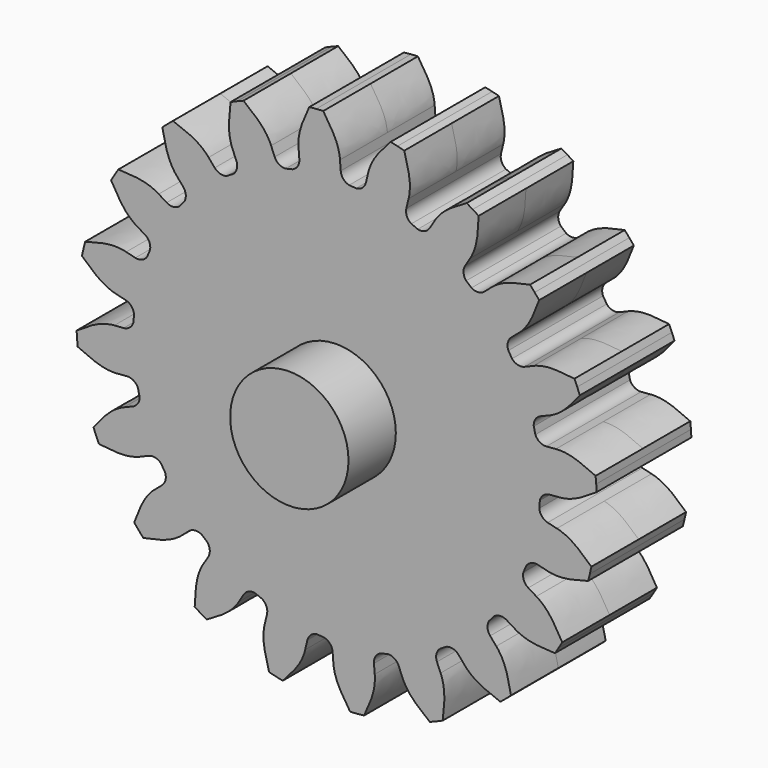
from build123d import *

# Parameters (mm, degrees)
F2_R     = 8.6
F3_DEPTH = 2.5
F5_DEPTH = 2.5
F6_COUNT = 20
F7_R     = 2.5
F8_DEPTH = 5


with BuildPart() as f3:
    # F2 (on Front) → F3 (new body, symmetric)
    with BuildSketch(Plane.XZ):
        Circle(F2_R)
    extrude(amount=F3_DEPTH, both=True)

    # F4 (on Front) → F5 (join, symmetric)
    with BuildSketch(Plane.XZ):
        with BuildLine():
            add(Edge.make_bspline(
                [(-0.5674598018, 10.9853534023), (-0.3230094132, 10.6269158767), (0.0665839323, 9.9930369158), (0.138145195, 9.4700722496), (0.1396836114, 9.4101594895), (0.1400502101, 9.3958825075)],
                knots=[0.2279557905, 0.2279557905, 0.2279557905, 0.2279557905, 0.5881424243, 0.9018559117, 1, 1, 1, 1], degree=3))
            ThreePointArc((-0.5674598018, 10.9853534023), (-0.7153197707, 10.9767170696), (-0.863050053, 10.9660906711))
            ThreePointArc((-0.863050053, 10.9660906711), (-1.0106238653, 10.9534761333), (-1.1580144527, 10.9388757433))
            add(Edge.make_bspline(
                [(-1.1580144527, 10.9388757433), (-1.3433832688, 10.5466107126), (-1.6290195576, 9.859590027), (-1.6178900847, 9.3318692759), (-1.61003714, 9.2724534799), (-1.6081658133, 9.2582949226)],
                knots=[0.2279557905, 0.2279557905, 0.2279557905, 0.2279557905, 0.5881424243, 0.9018559117, 1, 1, 1, 1], degree=3))
            Line((-1.6081658133, 9.2582949226), (-1.5768808199, 8.8607813922))
            ThreePointArc((-1.5768808199, 8.8607813922), (-1.6443578751, 8.5814007024), (-1.8636720345, 8.3956373521))
            ThreePointArc((-1.8636720345, 8.3956373521), (-1.272321563, 8.505362887), (-0.6747482233, 8.5734890701))
            ThreePointArc((-0.6747482233, 8.5734890701), (-0.0738747199, 8.5996826991), (0.5273601013, 8.5838156623))
            ThreePointArc((0.5273601013, 8.5838156623), (0.2816862729, 8.7329836642), (0.1713352034, 8.9983689771))
            Line((0.1713352034, 8.9983689771), (0.1400502101, 9.3958825075))
        make_face()
    extrude(amount=F5_DEPTH, both=True)

    # F6: F3 ×20 about axis
    f6_axis = Axis((0, -2.5, 0), (0, 1, 0))


with BuildPart() as f3_1:
    add(f3.part)
    for i in range(1, F6_COUNT):
        add(f3.part.rotate(f6_axis, i * 360 / F6_COUNT))

    # F7 (on Front) → F8 (join, symmetric)
    with BuildSketch(Plane.XZ):
        Circle(F7_R)
    extrude(amount=F8_DEPTH, both=True)


solid = f3_1.part
